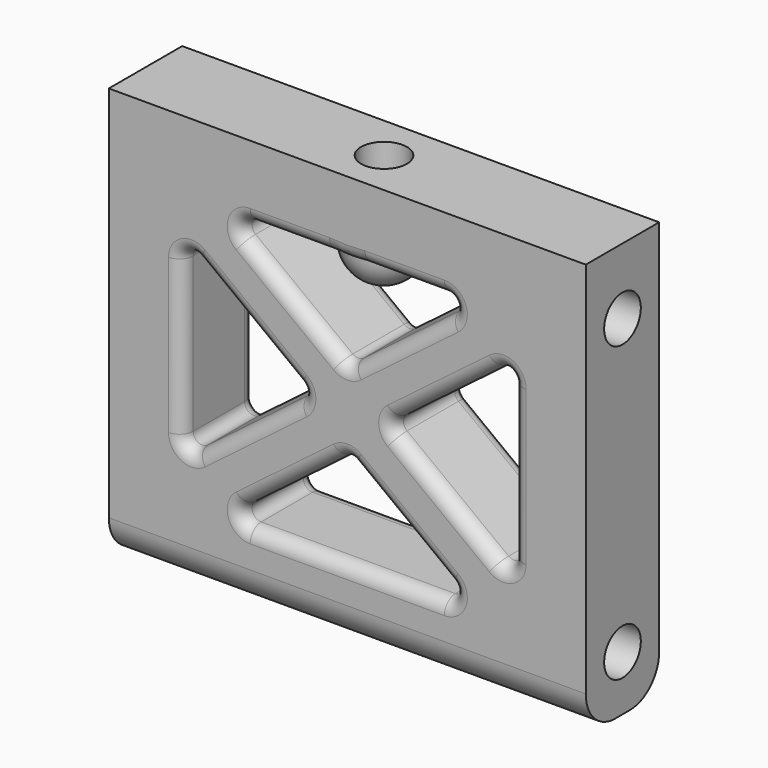
from build123d import *

# Parameters (mm, degrees)
F0_W     = 26
F0_H     = 22.6
F1_DEPTH = 5
F3_R     = 1.25
F4_DEPTH = 6
F2_R     = 1.25
F5_DEPTH = 6
F6_R     = 2
F7_DEPTH = 2
F8_R     = 1.25
F9_DEPTH = 5
F10_R    = 1.99999
F11_R    = 0.75
F12_R    = 2
F13_R    = 2


# Not quite as in the source:
# - a fillet or chamfer is up to 0.001 mm smaller than in the source, because OpenCascade refuses the exact size


with BuildPart() as f1:
    # F0 (on Front) → F1 (new body)
    with BuildSketch(Plane.XZ):
        with Locations((-39.6582745016, 37.2378250399)):
            Rectangle(F0_W, F0_H)
        with BuildLine():
            ThreePointArc((-34.0620873595, 30.8360469867), (-33.8905707158, 30.2783116759), (-34.364443575, 29.9378250399))
            Line((-34.364443575, 29.9378250399), (-44.9521054281, 29.9378250399))
            ThreePointArc((-44.9521054281, 29.9378250399), (-45.4259782873, 30.2783116759), (-45.2544616436, 30.8360469867))
            Line((-45.2544616436, 30.8360469867), (-39.9606307171, 34.8554705698))
            ThreePointArc((-39.9606307171, 34.8554705698), (-39.6582745016, 34.957248623), (-39.3559182861, 34.8554705698))
            Line((-39.3559182861, 34.8554705698), (-34.0620873595, 30.8360469867))
        make_face(mode=Mode.SUBTRACT)
        with BuildLine():
            ThreePointArc((-47.8559182861, 32.6840836764), (-48.3805602324, 32.6344339297), (-48.6582745016, 33.0823056232))
            Line((-48.6582745016, 33.0823056232), (-48.6582745016, 41.4933444566))
            ThreePointArc((-48.6582745016, 41.4933444566), (-48.3805602324, 41.9412161501), (-47.8559182861, 41.8915664034))
            Line((-47.8559182861, 41.8915664034), (-42.3169875687, 37.6860469867))
            ThreePointArc((-42.3169875687, 37.6860469867), (-42.1193437842, 37.2878250399), (-42.3169875687, 36.889603093))
            Line((-42.3169875687, 36.889603093), (-47.8559182861, 32.6840836764))
        make_face(mode=Mode.SUBTRACT)
        with BuildLine():
            Line((-30.6582745016, 41.4933444566), (-30.6582745016, 33.0823056232))
            ThreePointArc((-30.6582745016, 33.0823056232), (-30.9359887707, 32.6344339297), (-31.4606307171, 32.6840836764))
            Line((-31.4606307171, 32.6840836764), (-36.9995614344, 36.889603093))
            ThreePointArc((-36.9995614344, 36.889603093), (-37.1972052189, 37.2878250399), (-36.9995614344, 37.6860469867))
            Line((-36.9995614344, 37.6860469867), (-31.4606307171, 41.8915664034))
            ThreePointArc((-31.4606307171, 41.8915664034), (-30.9359887707, 41.9412161501), (-30.6582745016, 41.4933444566))
        make_face(mode=Mode.SUBTRACT)
        with BuildLine():
            Line((-44.9521054281, 44.5378250399), (-34.364443575, 44.5378250399))
            ThreePointArc((-34.364443575, 44.5378250399), (-33.8905707158, 44.1973384039), (-34.0620873595, 43.639603093))
            Line((-34.0620873595, 43.639603093), (-39.3559182861, 39.62017951))
            ThreePointArc((-39.3559182861, 39.62017951), (-39.6582745016, 39.5184014568), (-39.9606307171, 39.62017951))
            Line((-39.9606307171, 39.62017951), (-45.2544616436, 43.639603093))
            ThreePointArc((-45.2544616436, 43.639603093), (-45.4259782873, 44.1973384039), (-44.9521054281, 44.5378250399))
        make_face(mode=Mode.SUBTRACT)
    extrude(amount=F1_DEPTH)

    # F3 (on face) → F4 (cut)
    with BuildSketch(Plane(origin=(-52.6582745016, 0, 0), x_dir=(0, -1, 0), z_dir=(-1, 0, 0))):
        with Locations((2.5, 28.9378250399)):
            Circle(F3_R)
        with Locations((2.5, 44.9378250399)):
            Circle(F3_R)
    extrude(amount=-F4_DEPTH, mode=Mode.SUBTRACT)

    # F2 (on face) → F5 (cut)
    with BuildSketch(Plane.YZ.offset(-26.6582745016)):
        with Locations((-2.5, 28.9378250399)):
            Circle(F2_R)
        with Locations((-2.5, 44.9378250399)):
            Circle(F2_R)
    extrude(amount=-F5_DEPTH, mode=Mode.SUBTRACT)

    # F6 (on face) → F7 (join)
    with BuildSketch(Plane(origin=(0, 0, 44.5378250399), x_dir=(1, 0, 0), z_dir=(0, 0, -1))):
        with Locations((-39.6582745016, 2.5)):
            Circle(F6_R)
    extrude(amount=F7_DEPTH)

    # F8 (on face) → F9 (cut)
    with BuildSketch(Plane.XY.offset(48.5378250399)):
        with Locations((-39.6582745016, -2.5)):
            Circle(F8_R)
    extrude(amount=-F9_DEPTH, mode=Mode.SUBTRACT)

    # F10 (radius 2 in the source; OpenCascade refuses exactly that, so slightly less here)
    f10_edges = [f1.edges().sort_by_distance(p)[0] for p in [
        (-41.658275, -2.5, 42.537825),
    ]]
    fillet(f10_edges, radius=F10_R)

    # F11
    f11_edges = [f1.edges().sort_by_distance(p)[0] for p in [
        (-39.658275, 0, 44.537825),
        (-34.230096, 0, 34.786843),
        (-39.658275, 0, 29.937825),
        (-48.658275, 0, 37.287825),
        (-39.658275, -5, 29.937825),
        (-30.658275, -5, 37.287825),
        (-45.086453, -5, 34.786843),
        (-36.709003, -5, 41.629891),
    ]]
    fillet(f11_edges, radius=F11_R)

    # F12
    f12_edges = [f1.edges().sort_by_distance(p)[0] for p in [
        (-39.658275, 0, 25.937825),
    ]]
    fillet(f12_edges, radius=F12_R)

    # F13
    f13_edges = [f1.edges().sort_by_distance(p)[0] for p in [
        (-39.658275, -5, 25.937825),
    ]]
    fillet(f13_edges, radius=F13_R)


solid = f1.part
